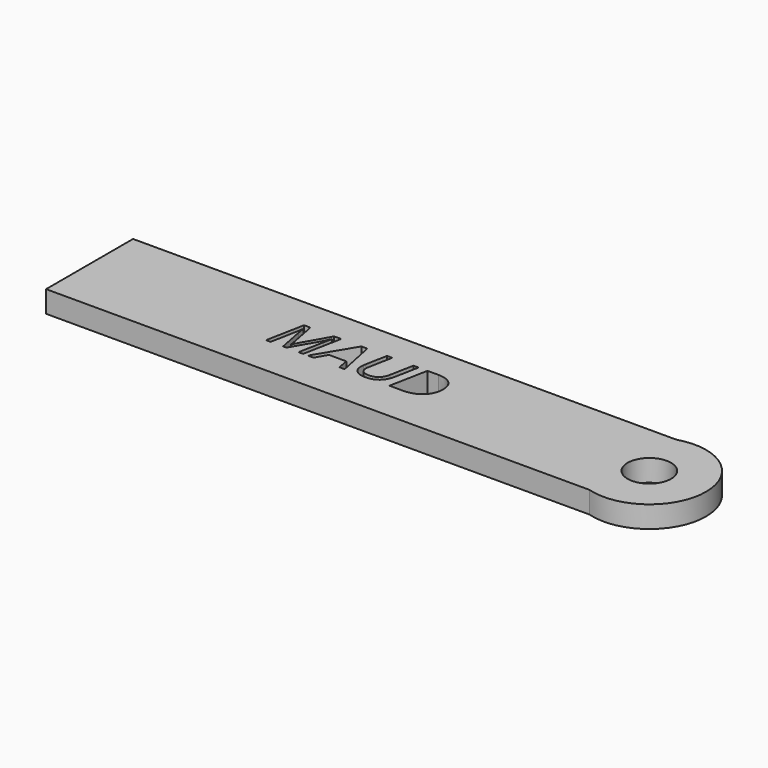
from build123d import *

# Parameters (mm, degrees)
F0_R     = 2
F1_DEPTH = 2


with BuildPart() as f1:
    # F0 (on Top) → F1 (new body)
    with BuildSketch(Plane.XY):
        with BuildLine():
            Line((15.6879561022, 26.1114555106), (-34.3120438978, 26.1114555106))
            Line((-34.3120438978, 26.1114555106), (-34.3120438978, 16.1114555106))
            Line((-34.3120438978, 16.1114555106), (15.6879561022, 16.1114555106))
            ThreePointArc((15.6879561022, 16.1114555106), (22.4158513012, 21.1114555106), (15.6879561022, 26.1114555106))
        make_face()
        with Locations((17.1939675076, 21.1114555106)):
            Circle(F0_R, mode=Mode.SUBTRACT)
        with BuildLine():
            Line((-13.594810762, 19.7880361229), (-14.0235288377, 19.7880361229))
            Line((-14.0235288377, 19.7880361229), (-13.5748518199, 22.1032734035))
            add(Edge.make_bspline(
                [(-13.5748518199, 22.1032734035), (-13.4846374017, 22.5647241443), (-13.4127852103, 22.8521329102)],
                knots=[0, 0, 0, 1, 1, 1], degree=2))
            add(Edge.make_bspline(
                [(-13.4127852103, 22.8521329102), (-13.6395187922, 22.3803035195), (-13.7744412407, 22.1535699376)],
                knots=[0, 0, 0, 1, 1, 1], degree=2))
            Line((-13.7744412407, 22.1535699376), (-15.1412295939, 19.7880361229))
            Line((-15.1412295939, 19.7880361229), (-15.4509923749, 19.7880361229))
            Line((-15.4509923749, 19.7880361229), (-15.9124431157, 22.1535699376))
            add(Edge.make_bspline(
                [(-15.9124431157, 22.1535699376), (-15.9276119116, 22.225422129), (-16.0146328991, 22.8521329102)],
                knots=[0, 0, 0, 1, 1, 1], degree=2))
            add(Edge.make_bspline(
                [(-16.0146328991, 22.8521329102), (-16.0369869142, 22.7020416658), (-16.0892793424, 22.3838961291)],
                knots=[0, 0, 0, 1, 1, 1], degree=2))
            add(Edge.make_bspline(
                [(-16.0892793424, 22.3838961291), (-16.1415717707, 22.0657505924), (-16.5886520731, 19.7880361229)],
                knots=[0, 0, 0, 1, 1, 1], degree=2))
            Line((-16.5886520731, 19.7880361229), (-17.0125800028, 19.7880361229))
            Line((-17.0125800028, 19.7880361229), (-16.3315808992, 23.3032050011))
            Line((-16.3315808992, 23.3032050011), (-15.7423929292, 23.3032050011))
            Line((-15.7423929292, 23.3032050011), (-15.2713618962, 20.8658189949))
            add(Edge.make_bspline(
                [(-15.2713618962, 20.8658189949), (-15.2514029542, 20.7684193576), (-15.1915261279, 20.3540717201)],
                knots=[0, 0, 0, 1, 1, 1], degree=2))
            Line((-15.1915261279, 20.3540717201), (-14.932059881, 20.885777937))
            Line((-14.932059881, 20.885777937), (-13.5524978048, 23.3032050011))
            Line((-13.5524978048, 23.3032050011), (-12.9138116584, 23.3032050011))
            Line((-12.9138116584, 23.3032050011), (-13.594810762, 19.7880361229))
        make_face(mode=Mode.SUBTRACT)
        Polygon((-9.7802577527, 19.7880361229), (-10.2664575817, 19.7880361229), (-10.4540716372, 20.8163208186), (-12.0483919301, 20.8163208186), (-12.6471601923, 19.7880361229), (-13.1660926862, 19.7880361229), (-11.0504448263, 23.3032050011), (-10.5083599596, 23.3032050011), align=None, mode=Mode.SUBTRACT)
        with BuildLine():
            add(Edge.make_bspline(
                [(-6.7688525726, 20.0834284656), (-7.1879903561, 19.7377395889), (-7.8737796058, 19.7377395889)],
                knots=[0, 0, 0, 1, 1, 1], degree=2))
            add(Edge.make_bspline(
                [(-7.8737796058, 19.7377395889), (-8.454983999, 19.7377395889), (-8.7894958682, 20.0387204354)],
                knots=[0, 0, 0, 1, 1, 1], degree=2))
            add(Edge.make_bspline(
                [(-8.7894958682, 20.0387204354), (-9.1240077373, 20.3397012819), (-9.1240077373, 20.8634239219)],
                knots=[0, 0, 0, 1, 1, 1], degree=2))
            add(Edge.make_bspline(
                [(-9.1240077373, 20.8634239219), (-9.1240077373, 20.9727989245), (-9.1052463318, 21.1264827784)],
                knots=[0, 0, 0, 1, 1, 1], degree=2))
            add(Edge.make_bspline(
                [(-9.1052463318, 21.1264827784), (-9.0864849262, 21.2801666324), (-9.0665259842, 21.3719777659)],
                knots=[0, 0, 0, 1, 1, 1], degree=2))
            Line((-9.0665259842, 21.3719777659), (-8.6920962308, 23.3032050011))
            Line((-8.6920962308, 23.3032050011), (-8.2154766941, 23.3032050011))
            Line((-8.2154766941, 23.3032050011), (-8.6202440394, 21.2003308641))
            add(Edge.make_bspline(
                [(-8.6202440394, 21.2003308641), (-8.6625569966, 20.9831775743), (-8.6625569966, 20.8434649798)],
                knots=[0, 0, 0, 1, 1, 1], degree=2))
            add(Edge.make_bspline(
                [(-8.6625569966, 20.8434649798), (-8.6625569966, 20.5041629645), (-8.4442061703, 20.3145530148)],
                knots=[0, 0, 0, 1, 1, 1], degree=2))
            add(Edge.make_bspline(
                [(-8.4442061703, 20.3145530148), (-8.225855344, 20.1249430651), (-7.8338617216, 20.1249430651)],
                knots=[0, 0, 0, 1, 1, 1], degree=2))
            add(Edge.make_bspline(
                [(-7.8338617216, 20.1249430651), (-6.8758325021, 20.1249430651), (-6.6842266582, 21.1380589648)],
                knots=[0, 0, 0, 1, 1, 1], degree=2))
            Line((-6.6842266582, 21.1380589648), (-6.2650888746, 23.3032050011))
            Line((-6.2650888746, 23.3032050011), (-5.7908644109, 23.3032050011))
            Line((-5.7908644109, 23.3032050011), (-6.2147923406, 21.1101164459))
            add(Edge.make_bspline(
                [(-6.2147923406, 21.1101164459), (-6.349714789, 20.4291173423), (-6.7688525726, 20.0834284656)],
                knots=[0, 0, 0, 1, 1, 1], degree=2))
        make_face(mode=Mode.SUBTRACT)
        with BuildLine():
            Line((-4.977337932, 23.3032050011), (-3.9594318862, 23.3032050011))
            add(Edge.make_bspline(
                [(-3.9594318862, 23.3032050011), (-3.1810331453, 23.3032050011), (-2.7355495582, 22.892849152)],
                knots=[0, 0, 0, 1, 1, 1], degree=2))
            add(Edge.make_bspline(
                [(-2.7355495582, 22.892849152), (-2.2900659711, 22.482493303), (-2.2900659711, 21.7615763152)],
                knots=[0, 0, 0, 1, 1, 1], degree=2))
            add(Edge.make_bspline(
                [(-2.2900659711, 21.7615763152), (-2.2900659711, 21.1723883452), (-2.547137145, 20.7308965465)],
                knots=[0, 0, 0, 1, 1, 1], degree=2))
            add(Edge.make_bspline(
                [(-2.547137145, 20.7308965465), (-2.8042083189, 20.2894047478), (-3.2868155383, 20.0387204354)],
                knots=[0, 0, 0, 1, 1, 1], degree=2))
            add(Edge.make_bspline(
                [(-3.2868155383, 20.0387204354), (-3.7694227576, 19.7880361229), (-4.3809647428, 19.7880361229)],
                knots=[0, 0, 0, 1, 1, 1], degree=2))
            Line((-4.3809647428, 19.7880361229), (-5.6583370355, 19.7880361229))
            Line((-5.6583370355, 19.7880361229), (-4.977337932, 23.3032050011))
        make_face(mode=Mode.SUBTRACT)
    extrude(amount=F1_DEPTH)


solid = f1.part
